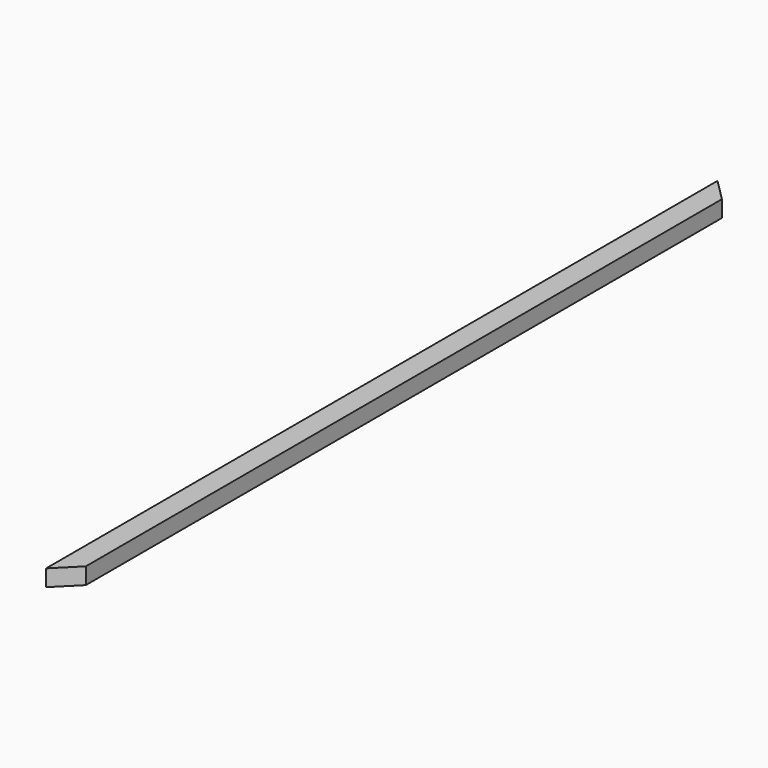
from build123d import *

# Parameters (mm, degrees)
F0_W     = 25.4
F0_H     = 965.2
F1_DEPTH = 19.05
F2_SIZE  = 25.39999


# Not quite as in the source:
# - a fillet or chamfer is up to 0.001 mm smaller than in the source, because OpenCascade refuses the exact size


with BuildPart() as f1:
    # F0 (on Top) → F1 (new body)
    with BuildSketch(Plane.XY):
        with Locations((-3.6795400083, 448.7868617729)):
            Rectangle(F0_W, F0_H)
    extrude(amount=F1_DEPTH)

    # F2 (size 25.4 in the source; OpenCascade refuses exactly that, so slightly less here)
    f2_edges = [f1.edges().sort_by_distance(p)[0] for p in [
        (9.02046, -33.813138, 9.525),
        (9.02046, 931.386862, 9.525),
    ]]
    chamfer(f2_edges, length=F2_SIZE)


solid = f1.part
